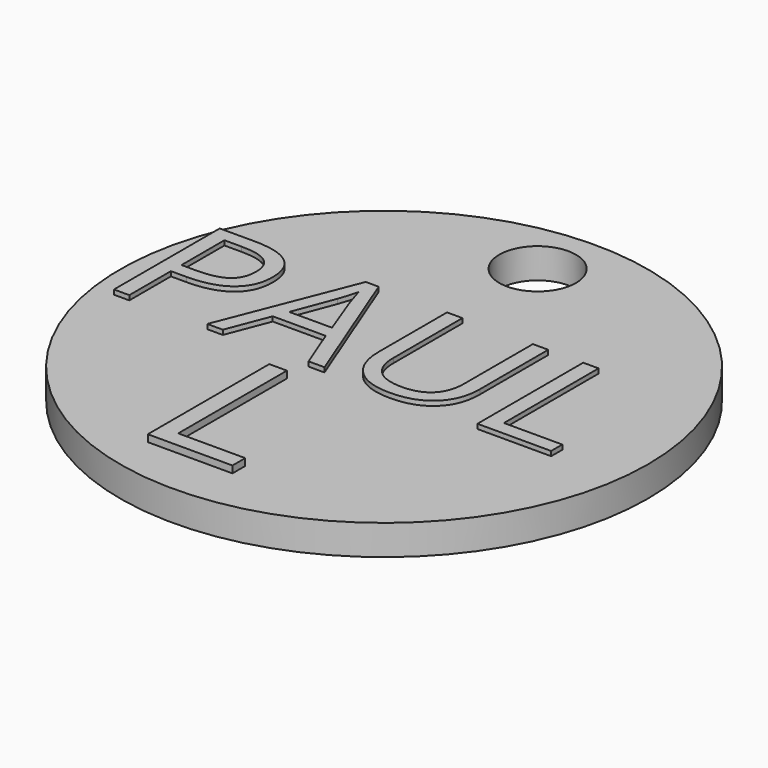
from build123d import *

# Parameters (mm, degrees)
F0_R         = 28.902306589
F1_DEPTH     = 3.302
F2_TEXT_SIZE = 20.2779297575
F3_DEPTH     = 3.81
F4_R         = 4.1991727701
F5_DEPTH     = 8.382
F6_TEXT_SIZE = 23.2889103548
F7_DEPTH     = 0.762


# Not quite as in the source:
# - Text() gives the source's letters only with a copy of the font that has no kerning and outlines rounded to 1/6400 em; it was checked with that copy


with BuildPart() as f1:
    # F0 (on Top) → F1 (new body)
    with BuildSketch(Plane.XY):
        Circle(F0_R)
    extrude(amount=F1_DEPTH)

    # F2 (on Top) → F3 (join)
    with BuildSketch(Plane.XY):
        with Locations((-28.3662066795, -4.0032473626)):
            Text('PAUL', F2_TEXT_SIZE, font='Open Sans', text_align=(TextAlign.LEFT, TextAlign.BOTTOM))
    extrude(amount=F3_DEPTH)

    # F4 (on Top) → F5 (cut)
    with BuildSketch(Plane.XY):
        with Locations((-1.0900765192, 22.3752651364)):
            Circle(F4_R)
    extrude(amount=F5_DEPTH, mode=Mode.SUBTRACT)

    # F6 (on face) → F7 (join)
    with BuildSketch(Plane.XY.offset(3.302)):
        with Locations((-9.3526439741, -23.5075522214)):
            Text('L', F6_TEXT_SIZE, font='Open Sans', text_align=(TextAlign.LEFT, TextAlign.BOTTOM))
    extrude(amount=F7_DEPTH)


solid = f1.part
